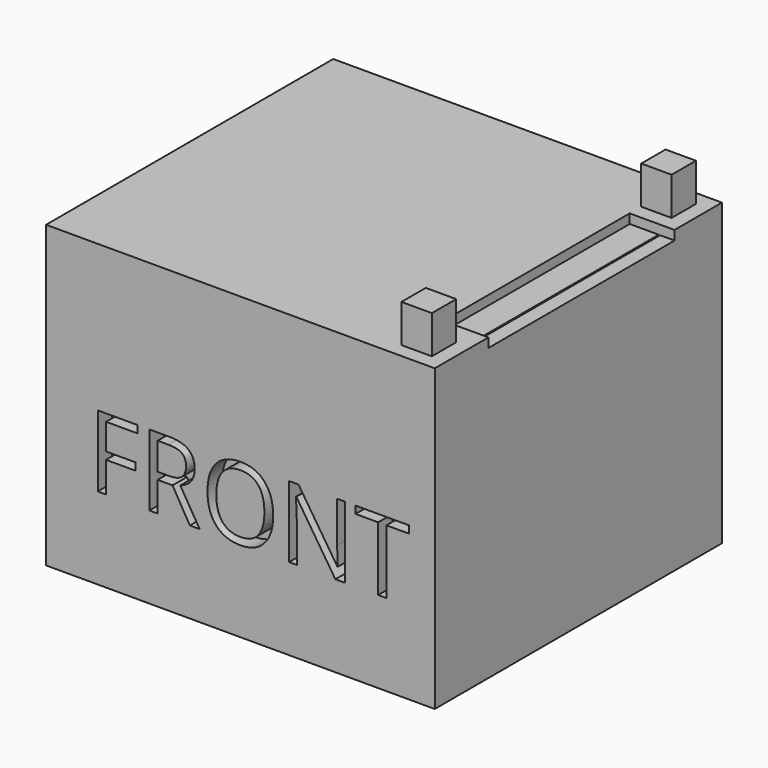
from build123d import *

# Parameters (mm, degrees)
F0_W         = 539.75
F0_H         = 498.45
F1_DEPTH     = 416.5
F2_TEXT_SIZE = 138.8888888889
F3_DEPTH     = 25
F4_W         = 42.2
F4_H         = 42.2
F5_DEPTH     = 52.8
F6_W         = 62.25
F6_H         = 323.1996848702
F7_DEPTH     = 13
F8_W         = 2
F8_H         = 323.1996848702
F9_DEPTH     = 5


# Not quite as in the source:
# - Text() gives the source's letters only with a copy of the font that has no kerning and outlines rounded to 1/6400 em; it was checked with that copy


with BuildPart() as f1:
    # F0 (on Top) → F1 (new body)
    with BuildSketch(Plane.XY):
        with Locations((269.875, 249.225)):
            Rectangle(F0_W, F0_H)
    extrude(amount=F1_DEPTH)

    # F2 (on face) → F3 (cut)
    with BuildSketch(Plane.XZ):
        with Locations((58.1273073968, 113.7937373559)):
            Text('FRONT', F2_TEXT_SIZE, font='Open Sans', text_align=(TextAlign.LEFT, TextAlign.BOTTOM))
    extrude(amount=-F3_DEPTH, mode=Mode.SUBTRACT)

    # F4 (on face) → F5 (join)
    with BuildSketch(Plane.XY.offset(416.5)):
        with Locations((498.6, 457.3)):
            Rectangle(F4_W, F4_H)
        with Locations((498.6, 41.15)):
            Rectangle(F4_W, F4_H)
    extrude(amount=F5_DEPTH)

    # F6 (on face) → F7 (cut)
    with BuildSketch(Plane.XY.offset(416.5)):
        with Locations((508.625, 254.6001575649)):
            Rectangle(F6_W, F6_H)
    extrude(amount=-F7_DEPTH, mode=Mode.SUBTRACT)

    # F8 (on face) → F9 (cut)
    with BuildSketch(Plane.XY.offset(403.5)):
        with Locations((518.75, 254.6001575649)):
            Rectangle(F8_W, F8_H)
    extrude(amount=-F9_DEPTH, mode=Mode.SUBTRACT)


solid = f1.part
